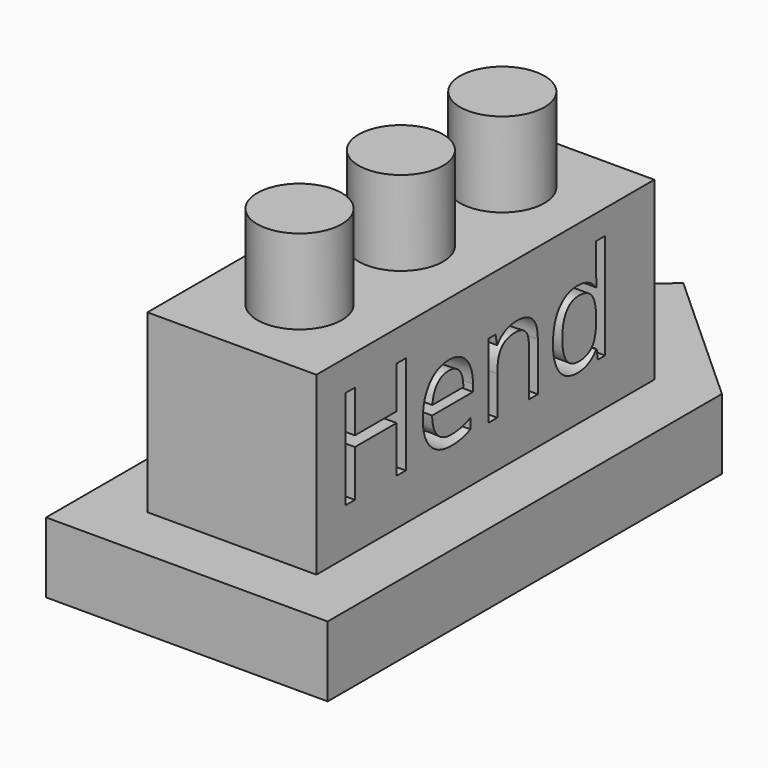
from build123d import *

# Parameters (mm, degrees)
F1_DEPTH     = 10
F2_W         = 24
F2_H         = 60
F3_DEPTH     = 25
F4_R         = 6
F5_DEPTH     = 12
F6_TEXT_SIZE = 19.671760189
F8_DEPTH     = 5
F7_TEXT_SIZE = 14.2296964062
F9_DEPTH     = 5


# Not quite as in the source:
# - Text() gives the source's letters only with a copy of the font that has no kerning and outlines rounded to 1/6400 em; it was checked with that copy


with BuildPart() as f1:
    # F0 (on Top) → F1 (new body)
    with BuildSketch(Plane.XY):
        Polygon((-16.6839058697, 50.6630543058), (-36.6839058697, 32.5246971586), (-36.6839058697, -37.4753028414), (3.3160941303, -37.4753028414), (3.3160941303, 32.5246971586), align=None)
    extrude(amount=F1_DEPTH)

    # F2 (on face) → F3 (join)
    with BuildSketch(Plane.XY.offset(10)):
        with Locations((-16.6839058697, 0.5246971586)):
            Rectangle(F2_W, F2_H)
    extrude(amount=F3_DEPTH)

    # F4 (on face) → F5 (join)
    with BuildSketch(Plane.XY.offset(35)):
        with Locations((-16.6839058697, 18.5246971586)):
            Circle(F4_R)
        with Locations((-16.6839058697, 0.5246971586)):
            Circle(F4_R)
        with Locations((-16.6839058697, -17.4753028414)):
            Circle(F4_R)
    extrude(amount=F5_DEPTH)

    # F6 (on face) → F8 (cut)
    with BuildSketch(Plane.YZ.offset(-4.6839058697)):
        with Locations((-26.2027885765, 16.5714938194)):
            Text('Hend', F6_TEXT_SIZE, font='Open Sans', text_align=(TextAlign.LEFT, TextAlign.BOTTOM))
    extrude(amount=-F8_DEPTH, mode=Mode.SUBTRACT)

    # F7 (on face) → F9 (cut)
    with BuildSketch(Plane(origin=(-28.6839058697, 0, 0), x_dir=(0, -1, 0), z_dir=(-1, 0, 0))):
        with Locations((-27.8373871782, 18.2159122988)):
            Text('Alanoud', F7_TEXT_SIZE, font='Open Sans', text_align=(TextAlign.LEFT, TextAlign.BOTTOM))
    extrude(amount=-F9_DEPTH, mode=Mode.SUBTRACT)


solid = f1.part
